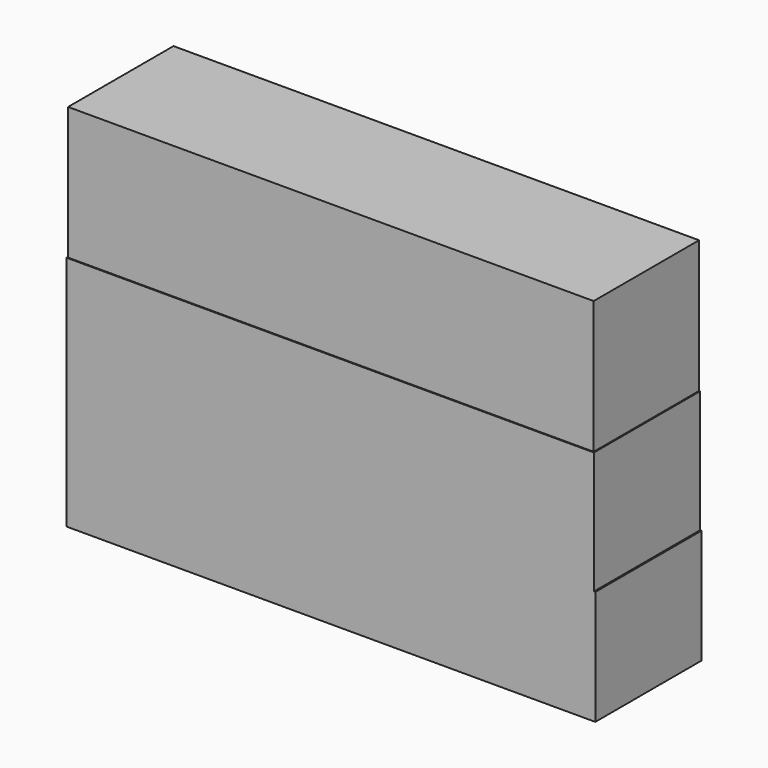
from build123d import *

# Parameters (mm, degrees)
F2_W     = 100.6348691881
F2_H     = 25.2255089581
F3_DEPTH = 25.4
F4_W     = 100.976370275
F4_H     = 23.4190355986
F5_DEPTH = 25.4
F8_W     = 101.243507117
F8_H     = 21.9049286097
F9_DEPTH = 25.4


# Not quite as in the source:
# - the program builds the solid bodies; features that only make, move or delete a surface that nothing else refers to are left out


with BuildPart() as f3:
    # F2 (on Top) → F3 (new body)
    with BuildSketch(Plane.XY):
        with Locations((-5.2274335176, -12.6127544791)):
            Rectangle(F2_W, F2_H)
    extrude(amount=F3_DEPTH)

    # F4 (on Front) → F5 (join)
    with BuildSketch(Plane.XZ):
        with Locations((-5.2071809769, -11.7095177993)):
            Rectangle(F4_W, F4_H)
    extrude(amount=F5_DEPTH)

    # F8 (on Front) → F9 (join)
    with BuildSketch(Plane.XZ):
        with Locations((-5.0736125559, -34.3714999035)):
            Rectangle(F8_W, F8_H)
    extrude(amount=F9_DEPTH)


solid = f3.part
